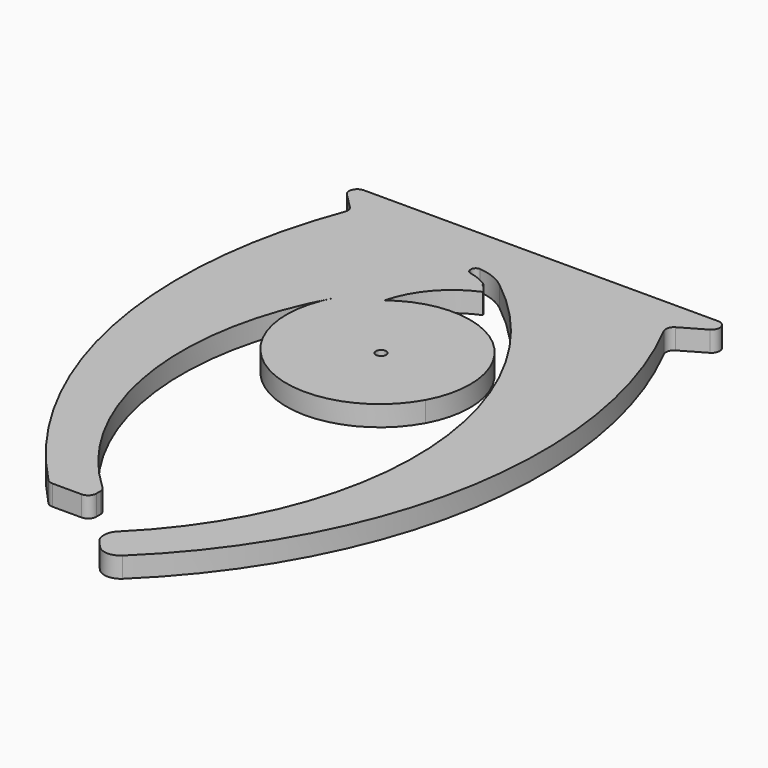
from build123d import *

# Parameters (mm, degrees)
F2_DEPTH  = 3.175
F1_R      = 13.594235125
F4_DEPTH  = 3.175
F6_DEPTH  = 3.175
F7_R      = 1.27
F8_R      = 0.762
F9_R      = 0.79375
F10_DEPTH = 3.176
F11_R     = 2.54


with BuildPart() as f2:
    # F1 (on face) → F2 (new body)
    with BuildSketch(Plane.XY):
        with BuildLine():
            Line((31.4070041795, 31.7847206253), (-31.4070041795, 31.7847206253))
            Line((-31.4070041795, 31.7847206253), (-26.3270041795, 26.7047206253))
            ThreePointArc((-26.3270041795, 26.7047206253), (-29.4018182362, -17.3120874939), (-6.8377400748, -55.230371411))
            Line((-6.8377400748, -55.230371411), (-2.5995985028, -50.5016658783))
            ThreePointArc((-2.5995985028, -50.5016658783), (-19.1698848855, -13.2713854087), (0, 22.6894778752))
            ThreePointArc((0, 22.6894778752), (20.2259208041, -17.2835334321), (2.6025941293, -58.4702772006))
            Line((2.6025941293, -58.4702772006), (6.8377400748, -63.2016658783))
            ThreePointArc((6.8377400748, -63.2016658783), (30.2976275511, -20.9804187613), (22.6081860771, 26.7047206253))
            Line((22.6081860771, 26.7047206253), (31.4070041795, 31.7847206253))
        make_face()
    extrude(amount=F2_DEPTH)



with BuildPart() as f2b:
    # F1 (on face) → F2, piece 2 (new body)
    with BuildSketch(Plane.XY):
        Circle(F1_R)
    extrude(amount=F2_DEPTH)


with BuildPart() as f2_1:
    add(f2.part)

    add(f2b.part)  # F4 merges F2b
    # F3 (on face) → F4 (join, through all)
    with BuildSketch(Plane.XY):
        with BuildLine():
            Line((-5.2498336251, 24.2303351167), (-13.4892699034, 7.3891431238))
            ThreePointArc((-13.4892699034, 7.3891431238), (-7.7433725843, -12.2768772355), (11.922647775, -6.5309799163))
            Line((11.922647775, -6.5309799163), (9.7925756653, -5.3641704599))
            ThreePointArc((9.7925756653, -5.3641704599), (-7.8384100149, 2.474239555), (0, 20.1052252351))
            Line((0, 20.1052252351), (-5.2498336251, 24.2303351167))
        make_face()
    extrude(amount=F4_DEPTH)

    # F5 (on face) → F6 (cut, through all)
    with BuildSketch(Plane.XY):
        Polygon((-3.9079916846, -49.3622544157), (-3.9079916846, -51.9615052849), (-10.2579916846, -51.9615052849), (-10.2579916846, -62.6840499783), (0, -56.9217726588), (-2.6145169004, -45.902473209), align=None)
        with BuildLine():
            Line((0, 19.5056907833), (0, 22.6894778752))
            ThreePointArc((0, 22.6894778752), (-2.5244121089, 24.0453912744), (-5.359141473, 24.4642791758))
            Line((-5.359141473, 24.4642791758), (-5.1168514161, 22.9205221383))
            ThreePointArc((-5.1168514161, 22.9205221383), (-3.237454866, 22.4415366371), (-1.5200501793, 21.5403820193))
            Line((-1.5200501793, 21.5403820193), (0, 19.5056907833))
        make_face()
    extrude(amount=F6_DEPTH, mode=Mode.SUBTRACT)

    # F7
    f7_edges = [f2_1.edges().sort_by_distance(p)[0] for p in [
        (-31.407004, 31.784721, 1.5875),
        (-26.327004, 26.704721, 1.5875),
        (31.407004, 31.784721, 1.5875),
        (22.608186, 26.704721, 1.5875),
        (-3.907992, -49.362254, 1.5875),
        (-3.907992, -51.961505, 1.5875),
        (-10.257992, -51.961505, 1.5875),
    ]]
    fillet(f7_edges, radius=F7_R)

    # F8
    f8_edges = [f2_1.edges().sort_by_distance(p)[0] for p in [
        (-5.359141, 24.464279, 1.5875),
        (-5.116851, 22.920522, 1.5875),
    ]]
    fillet(f8_edges, radius=F8_R)

    # F9 (on face) → F10 (cut, through all)
    with BuildSketch(Plane.XY.offset(3.175)):
        with Locations((0, -0.2915779182)):
            Circle(F9_R)
    extrude(amount=-F10_DEPTH, mode=Mode.SUBTRACT)

    # F11
    f11_edges = [f2_1.edges().sort_by_distance(p)[0] for p in [
        (2.602594, -58.470277, 1.5875),
        (6.83774, -63.201666, 1.5875),
    ]]
    fillet(f11_edges, radius=F11_R)


solid = f2_1.part
